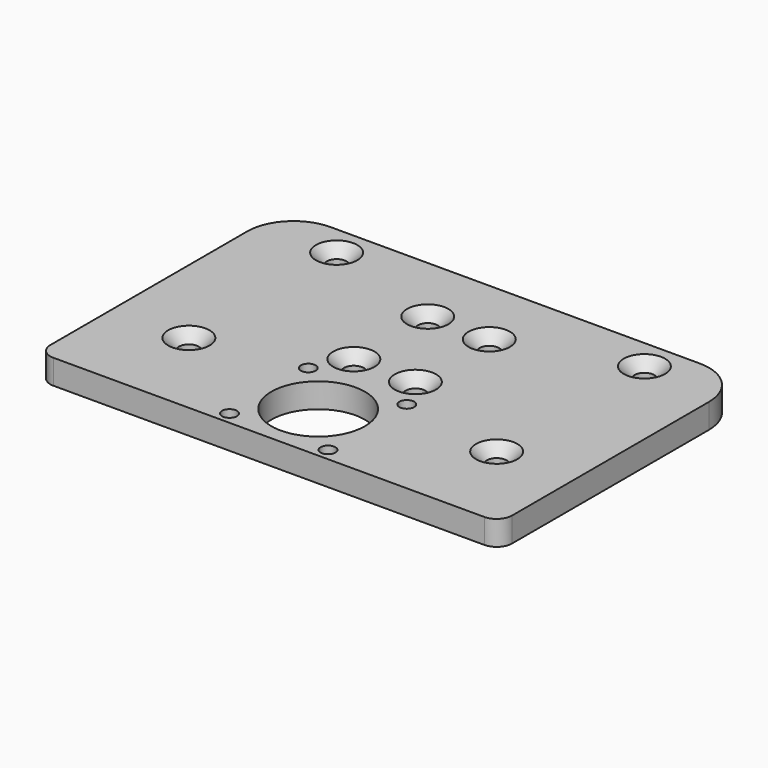
from build123d import *

# Parameters (mm, degrees)
F0_W           = 75
F0_H           = 50
F0_R           = 7.6
F1_DEPTH       = 4
F2_D           = 2.4
F3_D           = 3.2
F3_CSINK_D     = 6.72
F3_CSINK_ANGLE = 90
F4_R           = 7.5
F5_R           = 2.5


# Not quite as in the source:
# - a feature names something its author has since deleted; it is built from what else it names


with BuildPart() as f1:
    # F0 (on Top) → F1 (new body)
    with BuildSketch(Plane.XY):
        with Locations((0, 15)):
            Rectangle(F0_W, F0_H)
        Circle(F0_R, mode=Mode.SUBTRACT)
    extrude(amount=-F1_DEPTH)

    # F2 (through all)
    with Locations(Plane.XY):
        with Locations((-8, 8), (8, 8), (8, -8), (-8, -8)):
            Hole(F2_D / 2)

    # F3 (through all)
    with Locations(Plane.XY):
        with Locations((-25, 5), (25, 5), (-5, 28.5), (5, 28.5), (5, 13.5), (-5, 13.5), (-25, 35), (25, 35)):
            CounterSinkHole(F3_D / 2, F3_CSINK_D / 2, counter_sink_angle=F3_CSINK_ANGLE)

    # F4
    f4_edges = [f1.edges().sort_by_distance(p)[0] for p in [
        (-37.5, 40, -2),
        (37.5, 40, -2),
    ]]
    fillet(f4_edges, radius=F4_R)

    # F5
    f5_edges = [f1.edges().sort_by_distance(p)[0] for p in [
        (-37.5, -10, -2),
        (37.5, -10, -2),
    ]]
    fillet(f5_edges, radius=F5_R)


solid = f1.part
